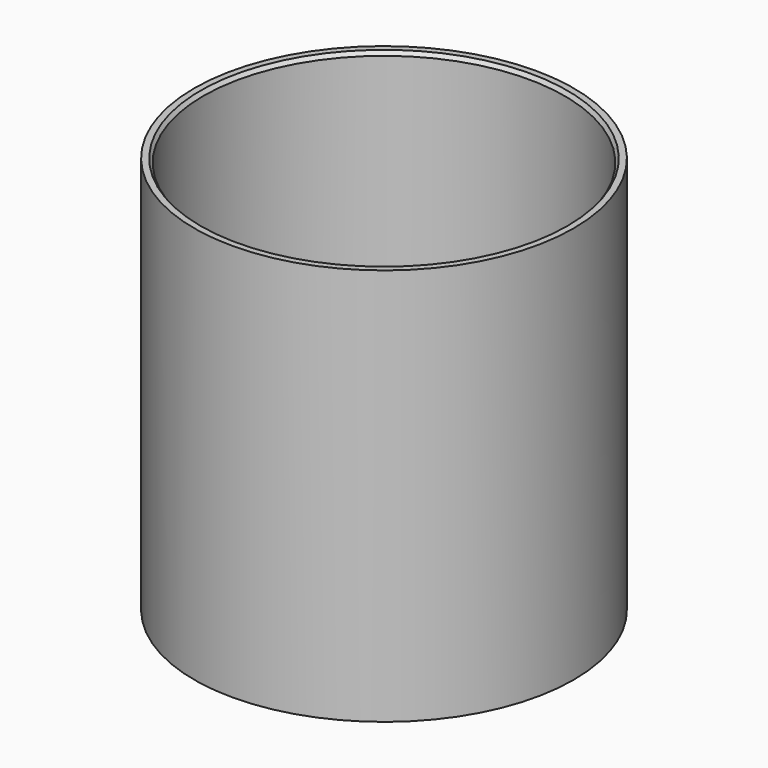
from build123d import *

# Parameters (mm, degrees)
F0_R       = 133.35
F0_R_2     = 127
F1_DEPTH   = 279.4
F5_SIZE2   = 2.7206219528
F5_SIZE    = 1.905
F5_2_SIZE2 = 2.7206219528
F5_2_SIZE  = 1.905


with BuildPart() as f1:
    # F0 (on Top) → F1 (new body)
    with BuildSketch(Plane.XY):
        Circle(F0_R)
        Circle(F0_R_2, mode=Mode.SUBTRACT)
    extrude(amount=F1_DEPTH)

    # F5
    f5_edges = [f1.edges().sort_by_distance(p)[0] for p in [
        (-127, 0, 279.4),
    ]]
    f5_side = f1.faces().sort_by_distance((-129.578292, 0, 279.4))[0]
    chamfer(f5_edges, length=F5_SIZE, length2=F5_SIZE2, reference=f5_side)

    # F5#2
    f5_2_edges = [f1.edges().sort_by_distance(p)[0] for p in [
        (-127, 0, 0),
    ]]
    f5_2_side = f1.faces().sort_by_distance((-129.578292, 0, 0))[0]
    chamfer(f5_2_edges, length=F5_2_SIZE, length2=F5_2_SIZE2, reference=f5_2_side)


solid = f1.part
